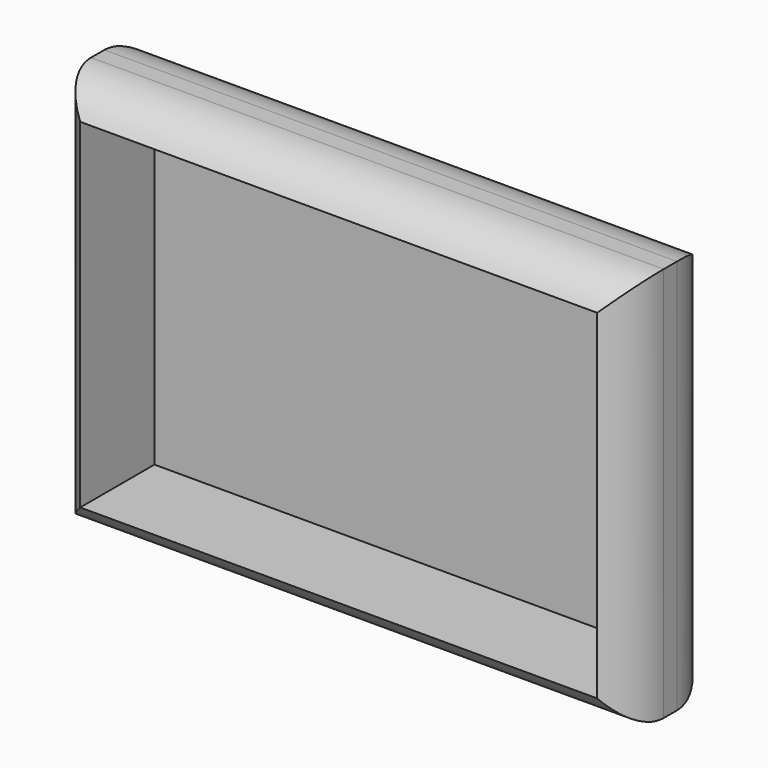
from build123d import *

# Parameters (mm, degrees)
F0_W        = 52.2474944592
F0_H        = 36.0527001321
F1_DEPTH    = 11.684
F2_T        = -2.54
F3_T1_DEPTH = 61.4527001321
F3_T3_DEPTH = 77.6474944592
F4_R        = 5.08


# Not quite as in the source:
# - a fillet or chamfer that OpenCascade refuses, or shapes differently, is made with other operations: its cross-section is extruded or revolved along the edge and cut away or added


with BuildPart() as f1:
    # F0 (on Front) → F1 (new body)
    with BuildSketch(Plane.XZ):
        with Locations((-5.1090717316, 18.0263500661)):
            Rectangle(F0_W, F0_H)
    extrude(amount=F1_DEPTH)

    # F2
    f2_openings = [f1.faces().sort_by_distance(p)[0] for p in [
        (-5.109072, -11.684, 18.02635),
    ]]
    offset(amount=F2_T, openings=f2_openings)

    # F3: fillet of radius 5.08 on 4 edges, made by hand

    # F3_s2 → F3_t1 (cut)
    with BuildSketch(Plane.XY.offset(-12.7)):
        with BuildLine():
            ThreePointArc((21.014675498, -6.604), (19.5267779464, -10.1961024484), (15.934675498, -11.684))
            Line((15.934675498, -11.684), (21.014675498, -11.684))
            Line((21.014675498, -11.684), (21.014675498, -6.604))
        make_face()
        with BuildLine():
            ThreePointArc((-31.2328189611, -6.604), (-29.7449214096, -10.1961024484), (-26.1528189611, -11.684))
            Line((-26.1528189611, -11.684), (-31.2328189611, -11.684))
            Line((-31.2328189611, -11.684), (-31.2328189611, -6.604))
        make_face()
    extrude(amount=F3_T1_DEPTH, mode=Mode.SUBTRACT)

    # F3_s4 → F3_t3 (cut)
    with BuildSketch(Plane.YZ.offset(-43.9328189611)):
        with BuildLine():
            ThreePointArc((-6.604, 36.0527001321), (-10.1961024484, 34.5648025806), (-11.684, 30.9727001321))
            Line((-11.684, 30.9727001321), (-11.684, 36.0527001321))
            Line((-11.684, 36.0527001321), (-6.604, 36.0527001321))
        make_face()
        with BuildLine():
            ThreePointArc((-6.604, 0), (-10.1961024484, 1.4878975516), (-11.684, 5.08))
            Line((-11.684, 5.08), (-11.684, 0))
            Line((-11.684, 0), (-6.604, 0))
        make_face()
    extrude(amount=F3_T3_DEPTH, mode=Mode.SUBTRACT)

    # F4
    f4_edges = [f1.edges().sort_by_distance(p)[0] for p in [
        (-5.109072, 0, 0),
        (-31.232819, 0, 18.02635),
        (-5.109072, 0, 36.0527),
        (21.014675, 0, 18.02635),
    ]]
    fillet(f4_edges, radius=F4_R)


solid = f1.part
